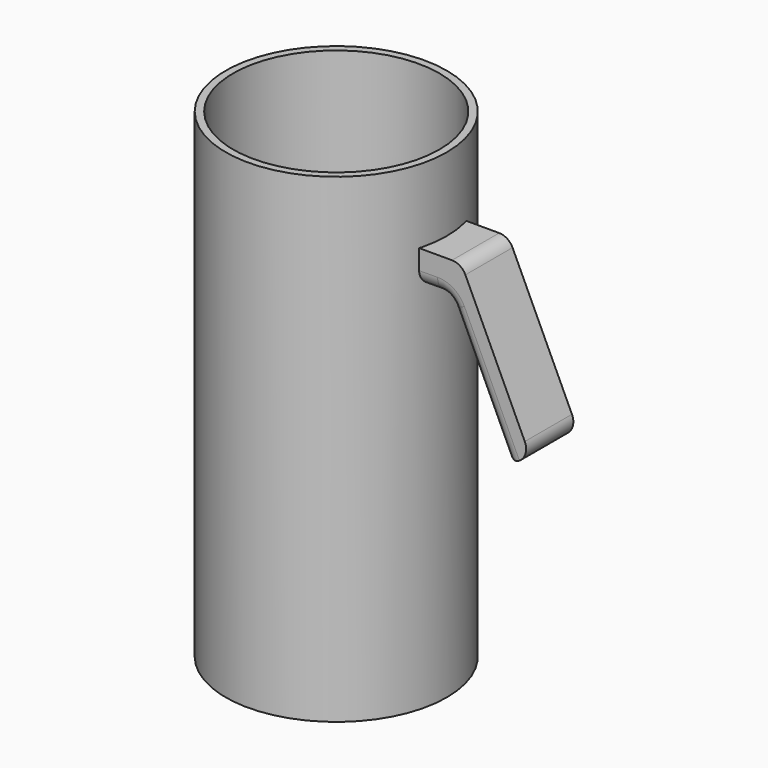
from build123d import *

# Parameters (mm, degrees)
F2_DEPTH    = 10.16
F3_R        = 5.08
F4_T        = -2.54
F5_R        = 5.08
F6_R        = 5.08
F7_T1_DEPTH = 59.8990400144
F9_T1_DEPTH = 52.7251544051
F9_T3_DEPTH = 19.9575926883
F9_T6_ANGLE = 65.45
F9_T8_ANGLE = 65.45


# Not quite as in the source:
# - a fillet or chamfer that OpenCascade refuses, or shapes differently, is made with other operations: its cross-section is extruded or revolved along the edge and cut away or added
# - a feature of the source that left no trace in its solid (it failed there, or was rolled back) is left out


with BuildPart() as f1:
    # F0 (on Front) → F1 (revolve)
    with BuildSketch(Plane.XZ):
        Polygon((19.8578521456, 79.4071055293), (-18.2421478544, 79.4071055293), (-18.2421478544, -85.9799182087), (19.8578521456, -85.9799182087), (19.8578521456, 42.1022108057), (17.5583876607, 42.0841504825), (17.5583876607, 54.0071055293), (19.8578521456, 54.0071055293), align=None)
        Polygon((19.8578521456, 42.1022108057), (19.8578521456, 54.0071055293), (17.5583876607, 54.0071055293), (17.5583876607, 42.0841504825), align=None)
    revolve(axis=Axis((-18.2421478544, 0, -3.2864063397), (0, 0, -1)))

    # F4
    f4_openings = [f1.faces().sort_by_distance(p)[0] for p in [
        (-18.242148, 0, 79.407106),
    ]]
    offset(amount=F4_T, openings=f4_openings)


with BuildPart() as f2:
    # F0 (on Front) → F2 (new body, symmetric)
    with BuildSketch(Plane.XZ):
        Polygon((33.0144607576, 54.0071055293), (19.8578521456, 54.0071055293), (19.8578521456, 42.1022108057), (28.0800888653, 42.1667894297), (47.7427856962, 0), (58.1983876607, 0), align=None)
        Polygon((19.8578521456, 42.1022108057), (19.8578521456, 54.0071055293), (17.5583876607, 54.0071055293), (17.5583876607, 42.0841504825), align=None)
    extrude(amount=F2_DEPTH, both=True)

    # F3
    f3_edges = [f2.edges().sort_by_distance(p)[0] for p in [
        (33.014461, 0, 54.007106),
    ]]
    fillet(f3_edges, radius=F3_R)

    # F5
    f5_edges = [f2.edges().sort_by_distance(p)[0] for p in [
        (28.080089, 0, 42.166789),
    ]]
    fillet(f5_edges, radius=F5_R)

    # F6
    f6_edges = [f2.edges().sort_by_distance(p)[0] for p in [
        (47.742786, 0, 0),
    ]]
    fillet(f6_edges, radius=F6_R)

    # F7: fillet of radius 5.08 on 1 edges, made by hand

    # F7_s2 → F7_t1 (cut)
    with BuildSketch(Plane.XZ.offset(-29.9495200072)):
        with BuildLine():
            ThreePointArc((50.9791026211, 0), (54.7189312044, 2.6135617341), (54.8530226422, 7.1741584337))
            Line((54.8530226422, 7.1741584337), (58.1983876607, 0))
            Line((58.1983876607, 0), (50.9791026211, 0))
        make_face()
    extrude(amount=F7_T1_DEPTH, mode=Mode.SUBTRACT)

    # F9: fillet of radius 5.08 on 6 edges, made by hand

    # F9_s2 → F9_t1 (cut)
    with BuildSketch(Plane(origin=(-9.7559305144, 0, 20.9216605042), x_dir=(0, 1, 0), z_dir=(0.4226182617, 0, -0.906307787))):
        with BuildLine():
            ThreePointArc((10.16, 48.3496584513), (8.6721024484, 44.7575560028), (5.08, 43.2696584513))
            Line((5.08, 43.2696584513), (10.16, 43.2696584513))
            Line((10.16, 43.2696584513), (10.16, 48.3496584513))
        make_face()
        with BuildLine():
            ThreePointArc((-5.08, 43.2696584513), (-8.6721024484, 44.7575560028), (-10.16, 48.3496584513))
            Line((-10.16, 48.3496584513), (-10.16, 43.2696584513))
            Line((-10.16, 43.2696584513), (-5.08, 43.2696584513))
        make_face()
    extrude(amount=F9_T1_DEPTH, mode=Mode.SUBTRACT)

    # F9_s4 → F9_t3 (cut)
    with BuildSketch(Plane(origin=(5.1882108439, 0, 0.0407489506), x_dir=(0, 1, 0), z_dir=(0.9999691576, 0, 0.0078539009))):
        with BuildLine():
            ThreePointArc((10.16, 47.0249506718), (8.6721024484, 43.4328482233), (5.08, 41.9449506718))
            Line((5.08, 41.9449506718), (10.16, 41.9449506718))
            Line((10.16, 41.9449506718), (10.16, 47.0249506718))
        make_face()
        with BuildLine():
            ThreePointArc((-5.08, 41.9449506718), (-8.6721024484, 43.4328482233), (-10.16, 47.0249506718))
            Line((-10.16, 47.0249506718), (-10.16, 41.9449506718))
            Line((-10.16, 41.9449506718), (-5.08, 41.9449506718))
        make_face()
    extrude(amount=F9_T3_DEPTH, mode=Mode.SUBTRACT)

    # F9_s5 → F9_t6 (revolve, cut)
    with BuildSketch(Plane(origin=(25.1451879931, 0, 0.1974939055), x_dir=(0, 1, 0), z_dir=(-0.9999691576, 0, -0.0078539009))):
        with BuildLine():
            ThreePointArc((10.16, -47.0249506718), (8.6721024484, -43.4328482233), (5.08, -41.9449506718))
            Line((5.08, -41.9449506718), (10.16, -41.9449506718))
            Line((10.16, -41.9449506718), (10.16, -47.0249506718))
        make_face()
    revolve(axis=Axis((24.8556543242, 10.16, 37.0613075754), (0, 1, 0)), revolution_arc=F9_T6_ANGLE, mode=Mode.SUBTRACT)

    # F9_s7 → F9_t8 (revolve, cut)
    with BuildSketch(Plane(origin=(25.1451879931, 0, 0.1974939055), x_dir=(0, 1, 0), z_dir=(-0.9999691576, 0, -0.0078539009))):
        with BuildLine():
            ThreePointArc((-5.08, -41.9449506718), (-8.6721024484, -43.4328482233), (-10.16, -47.0249506718))
            Line((-10.16, -47.0249506718), (-10.16, -41.9449506718))
            Line((-10.16, -41.9449506718), (-5.08, -41.9449506718))
        make_face()
    revolve(axis=Axis((24.8556543242, -10.16, 37.0613075754), (0, 1, 0)), revolution_arc=F9_T8_ANGLE, mode=Mode.SUBTRACT)


solid = Compound([f1.part, f2.part])
